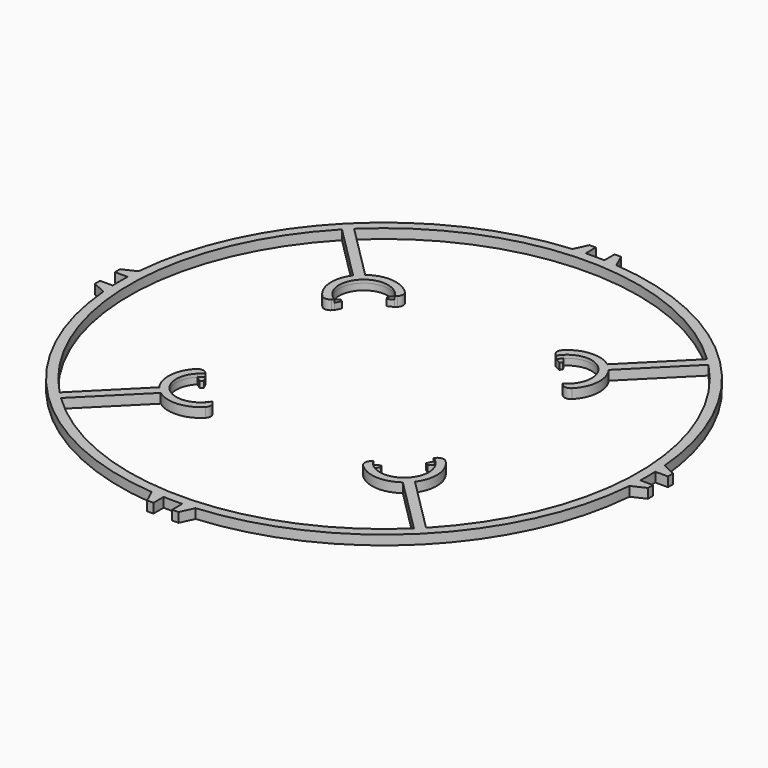
from build123d import *
from build123d import SkipClean  # not in build123d's __all__

# Parameters (mm, degrees)
F1_R     = 41.5
F2_DEPTH = 1.5
F3_R     = 3.85
F4_DEPTH = 0.5
F6_DEPTH = 1.5


with BuildPart() as f2:
    # F1 (on face) → F2 (new body)
    with BuildSketch(Plane.XY):
        Circle(F1_R)
        with BuildLine():
            ThreePointArc((-28.8093051541, -27.7493051541), (-40, 0), (-28.8093051541, 27.7493051541))
            Line((-28.8093051541, 27.7493051541), (-20.0970856452, 19.0370856452))
            ThreePointArc((-20.0970856452, 19.0370856452), (-21.086593154, 15.6304460992), (-19.6150738914, 12.4026063935))
            ThreePointArc((-19.6150738914, 12.4026063935), (-18.9074615459, 12.1079784401), (-18.1991290923, 12.4008709077))
            Line((-18.1991290923, 12.4008709077), (-17.9308268662, 12.6691731338))
            Line((-17.9308268662, 12.6691731338), (-17.4883090065, 13.565932825))
            Line((-17.4883090065, 13.565932825), (-17.9010595127, 13.8481331433))
            Line((-17.9010595127, 13.8481331433), (-18.7223611076, 13.2776388924))
            ThreePointArc((-18.7223611076, 13.2776388924), (-18.7223611076, 18.7223611076), (-13.2776388924, 18.7223611076))
            Line((-13.2776388924, 18.7223611076), (-13.8477912725, 17.9008221471))
            Line((-13.8477912725, 17.9008221471), (-13.5657589526, 17.4879568294))
            Line((-13.5657589526, 17.4879568294), (-12.6691731338, 17.9308268662))
            Line((-12.6691731338, 17.9308268662), (-12.4008709077, 18.1991290923))
            ThreePointArc((-12.4008709077, 18.1991290923), (-12.1079784401, 18.9074615459), (-12.4026063935, 19.6150738914))
            ThreePointArc((-12.4026063935, 19.6150738914), (-15.6304460992, 21.086593154), (-19.0370856452, 20.0970856452))
            Line((-19.0370856452, 20.0970856452), (-27.7493051541, 28.8093051541))
            ThreePointArc((-27.7493051541, 28.8093051541), (0, 40), (27.7493051541, 28.8093051541))
            Line((27.7493051541, 28.8093051541), (19.0370856452, 20.0970856452))
            ThreePointArc((19.0370856452, 20.0970856452), (15.6304460992, 21.086593154), (12.4026063935, 19.6150738914))
            ThreePointArc((12.4026063935, 19.6150738914), (12.1079784401, 18.9074615459), (12.4008709077, 18.1991290923))
            Line((12.4008709077, 18.1991290923), (12.6691731338, 17.9308268662))
            Line((12.6691731338, 17.9308268662), (13.565932825, 17.4883090065))
            Line((13.565932825, 17.4883090065), (13.8481331433, 17.9010595127))
            Line((13.8481331433, 17.9010595127), (13.2776388924, 18.7223611076))
            ThreePointArc((13.2776388924, 18.7223611076), (18.7223611076, 18.7223611076), (18.7223611076, 13.2776388924))
            Line((18.7223611076, 13.2776388924), (17.9008221471, 13.8477912725))
            Line((17.9008221471, 13.8477912725), (17.4879568294, 13.5657589526))
            Line((17.4879568294, 13.5657589526), (17.9308268662, 12.6691731338))
            Line((17.9308268662, 12.6691731338), (18.1991290923, 12.4008709077))
            ThreePointArc((18.1991290923, 12.4008709077), (18.9074615459, 12.1079784401), (19.6150738914, 12.4026063935))
            ThreePointArc((19.6150738914, 12.4026063935), (21.086593154, 15.6304460992), (20.0970856452, 19.0370856452))
            Line((20.0970856452, 19.0370856452), (28.8093051541, 27.7493051541))
            ThreePointArc((28.8093051541, 27.7493051541), (40, 0), (28.8093051541, -27.7493051541))
            Line((28.8093051541, -27.7493051541), (20.0970856452, -19.0370856452))
            ThreePointArc((20.0970856452, -19.0370856452), (21.086593154, -15.6304460992), (19.6150738914, -12.4026063935))
            ThreePointArc((19.6150738914, -12.4026063935), (18.9074615459, -12.1079784401), (18.1991290923, -12.4008709077))
            Line((18.1991290923, -12.4008709077), (17.9308268662, -12.6691731338))
            Line((17.9308268662, -12.6691731338), (17.4883090065, -13.565932825))
            Line((17.4883090065, -13.565932825), (17.9010595127, -13.8481331433))
            Line((17.9010595127, -13.8481331433), (18.7223611076, -13.2776388924))
            ThreePointArc((18.7223611076, -13.2776388924), (18.7223611076, -18.7223611076), (13.2776388924, -18.7223611076))
            Line((13.2776388924, -18.7223611076), (13.8477912725, -17.9008221471))
            Line((13.8477912725, -17.9008221471), (13.5657589526, -17.4879568294))
            Line((13.5657589526, -17.4879568294), (12.6691731338, -17.9308268662))
            Line((12.6691731338, -17.9308268662), (12.4008709077, -18.1991290923))
            ThreePointArc((12.4008709077, -18.1991290923), (12.1079784401, -18.9074615459), (12.4026063935, -19.6150738914))
            ThreePointArc((12.4026063935, -19.6150738914), (15.6304460992, -21.086593154), (19.0370856452, -20.0970856452))
            Line((19.0370856452, -20.0970856452), (27.7493051541, -28.8093051541))
            ThreePointArc((27.7493051541, -28.8093051541), (0, -40), (-27.7493051541, -28.8093051541))
            Line((-27.7493051541, -28.8093051541), (-19.0370856452, -20.0970856452))
            ThreePointArc((-19.0370856452, -20.0970856452), (-15.6304460992, -21.086593154), (-12.4026063935, -19.6150738914))
            ThreePointArc((-12.4026063935, -19.6150738914), (-12.1079784401, -18.9074615459), (-12.4008709077, -18.1991290923))
            Line((-12.4008709077, -18.1991290923), (-12.6691731338, -17.9308268662))
            Line((-12.6691731338, -17.9308268662), (-13.565932825, -17.4883090065))
            Line((-13.565932825, -17.4883090065), (-13.8481331433, -17.9010595127))
            Line((-13.8481331433, -17.9010595127), (-13.2776388924, -18.7223611076))
            ThreePointArc((-13.2776388924, -18.7223611076), (-18.7223611076, -18.7223611076), (-18.7223611076, -13.2776388924))
            Line((-18.7223611076, -13.2776388924), (-17.9008221471, -13.8477912725))
            Line((-17.9008221471, -13.8477912725), (-17.4879568294, -13.5657589526))
            Line((-17.4879568294, -13.5657589526), (-17.9308268662, -12.6691731338))
            Line((-17.9308268662, -12.6691731338), (-18.1991290923, -12.4008709077))
            ThreePointArc((-18.1991290923, -12.4008709077), (-18.9074615459, -12.1079784401), (-19.6150738914, -12.4026063935))
            ThreePointArc((-19.6150738914, -12.4026063935), (-21.086593154, -15.6304460992), (-20.0970856452, -19.0370856452))
            Line((-20.0970856452, -19.0370856452), (-28.8093051541, -27.7493051541))
        make_face(mode=Mode.SUBTRACT)
    extrude(amount=F2_DEPTH)

    # F3 (on face) → F4 (cut)
    with BuildSketch(Plane.XY.offset(1.5)):
        with Locations((-16, 16)):
            Circle(F3_R)
        with Locations((-16, -16)):
            Circle(F3_R)
        with Locations((16, -16)):
            Circle(F3_R)
        with Locations((16, 16)):
            Circle(F3_R)
    with SkipClean():  # cleaning this boolean's faces spoils the solid; the shape is the same uncleaned
        extrude(amount=-F4_DEPTH, mode=Mode.SUBTRACT)

    # F5 (on Top) → F6 (join)
    with BuildSketch(Plane.XY):
        Polygon((-1.47, 41.4739568886), (-1.47, 43.4739568886), (-2.47, 43.4739568886), (-3.4575279787, 41.3557190758), align=None)
        Polygon((2.47, 43.4739568886), (1.47, 43.4739568886), (1.47, 41.4739568886), (3.4575279787, 41.3557190758), align=None)
        Polygon((-43.4739568886, 2.47), (-43.4739568886, 1.47), (-41.4739568886, 1.47), (-41.3557190758, 3.4575279787), align=None)
        Polygon((-41.4739568886, -1.47), (-43.4739568886, -1.47), (-43.4739568886, -2.47), (-41.3557190758, -3.4575279787), align=None)
        Polygon((-2.47, -43.4739568886), (-1.47, -43.4739568886), (-1.47, -41.4739568886), (-3.4575279787, -41.3557190758), align=None)
        Polygon((1.47, -41.4739568886), (1.47, -43.4739568886), (2.47, -43.4739568886), (3.4575279787, -41.3557190758), align=None)
        Polygon((43.4739568886, -2.47), (43.4739568886, -1.47), (41.4739568886, -1.47), (41.3557190758, -3.4575279787), align=None)
        Polygon((41.4739568886, 1.47), (43.4739568886, 1.47), (43.4739568886, 2.47), (41.3557190758, 3.4575279787), align=None)
    extrude(amount=F6_DEPTH)


solid = f2.part
